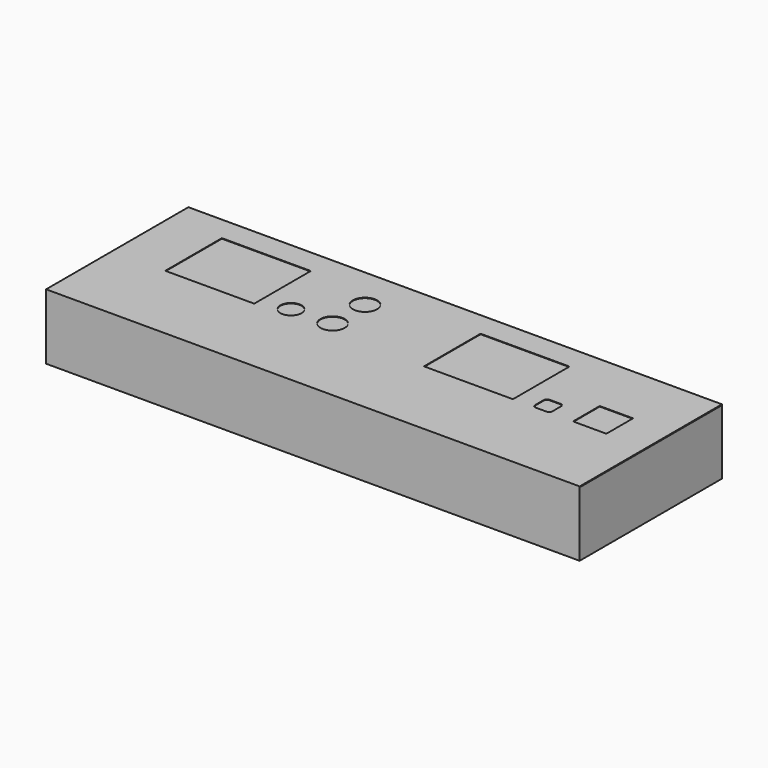
from build123d import *

# Parameters (mm, degrees)
F1_DEPTH = 209.55
F2_W     = 69.85
F2_H     = 55.5625
F2_W_2   = 26.19375
F2_H_2   = 26.19375
F3_DEPTH = 0.4064


# Not quite as in the source:
# - the dataset's text gives a spline's control points without its knots; the knots are read off the source's solid


with BuildPart() as f1:
    # F0 (on Right) → F1 (new body, symmetric)
    with BuildSketch(Plane.YZ):
        Polygon((-139.7, 0), (0, 0), (0, 50.8), (-139.2936, 50.8), (-139.2936, 51.054), (0, 51.054), (0, 51.4604), (-139.7, 51.4604), align=None)
    extrude(amount=F1_DEPTH, both=True)

    # F2 (on face) → F3 (cut, through all)
    with BuildSketch(Plane.XY.offset(51.4604)):
        with Locations((-132.8911783457, -47.0433160888)):
            Rectangle(F2_W, F2_H)
        with Locations((70.3088216543, -47.0433160888)):
            Rectangle(F2_W, F2_H)
        with BuildLine():
            add(Edge.make_bspline(
                [(121.4099132543, -62.0291382888), (120.9689438543, -62.4693964888), (120.7119466543, -63.0892072888), (120.7119466543, -63.7120660888)],
                knots=[1, 1, 1, 1, 2, 2, 2, 2], degree=3))
            Line((120.7119466543, -63.7120660888), (120.7119466543, -72.4433160888))
            add(Edge.make_bspline(
                [(120.7119466543, -72.4433160888), (120.7119466543, -73.0672416888), (120.9689438543, -73.6870016888), (121.4099132543, -74.1272598888)],
                knots=[0, 0, 0, 0, 1, 1, 1, 1], degree=3))
            add(Edge.make_bspline(
                [(121.4099132543, -74.1272598888), (121.8505270543, -74.5682292888), (122.4699822543, -74.8245660888), (123.0931966543, -74.8245660888)],
                knots=[1, 1, 1, 1, 2, 2, 2, 2], degree=3))
            Line((123.0931966543, -74.8245660888), (131.8244466543, -74.8245660888))
            add(Edge.make_bspline(
                [(131.8244466543, -74.8245660888), (132.4483468543, -74.8245660888), (133.0677766543, -74.5682292888), (133.5083904543, -74.1272598888)],
                knots=[0, 0, 0, 0, 1, 1, 1, 1], degree=3))
            add(Edge.make_bspline(
                [(133.5083904543, -74.1272598888), (133.9490042543, -73.6870016888), (134.2056966543, -73.0672416888), (134.2056966543, -72.4433160888)],
                knots=[1, 1, 1, 1, 2, 2, 2, 2], degree=3))
            Line((134.2056966543, -72.4433160888), (134.2056966543, -63.7120660888))
            add(Edge.make_bspline(
                [(134.2056966543, -63.7120660888), (134.2056966543, -63.0892072888), (133.9490042543, -62.4693964888), (133.5083904543, -62.0291382888)],
                knots=[0, 0, 0, 0, 1, 1, 1, 1], degree=3))
            add(Edge.make_bspline(
                [(133.5083904543, -62.0291382888), (133.0677766543, -61.5881688888), (132.4483468543, -61.3308160888), (131.8244466543, -61.3308160888)],
                knots=[1, 1, 1, 1, 2, 2, 2, 2], degree=3))
            Line((131.8244466543, -61.3308160888), (123.0931966543, -61.3308160888))
            add(Edge.make_bspline(
                [(123.0931966543, -61.3308160888), (122.4699822543, -61.3308160888), (121.8505270543, -61.5881688888), (121.4099132543, -62.0291382888)],
                knots=[0, 0, 0, 0, 1, 1, 1, 1], degree=3))
        make_face()
        with Locations((165.5588216543, -61.7276910888)):
            Rectangle(F2_W_2, F2_H_2)
        with BuildLine():
            add(Edge.make_bspline(
                [(-69.8476671457, -60.5980514888), (-71.3907171457, -59.0546712888), (-73.5590643457, -58.1558160888), (-75.7411783457, -58.1558160888)],
                knots=[7, 7, 7, 7, 8, 8, 8, 8], degree=3))
            add(Edge.make_bspline(
                [(-75.7411783457, -58.1558160888), (-77.9229621457, -58.1558160888), (-80.0913093457, -59.0546712888), (-81.6343593457, -60.5980514888)],
                knots=[0, 0, 0, 0, 1, 1, 1, 1], degree=3))
            add(Edge.make_bspline(
                [(-81.6343593457, -60.5980514888), (-83.1771045457, -62.1407712888), (-84.0755533457, -64.3087628888), (-84.0755533457, -66.4901910888), (-84.0755533457, -68.6726606888), (-83.1771045457, -70.8406522888), (-81.6343593457, -72.3840578888)],
                knots=[1, 1, 1, 1, 2, 2, 2, 3, 3, 3, 3], degree=3))
            add(Edge.make_bspline(
                [(-81.6343593457, -72.3840578888), (-80.0913093457, -73.9267776888), (-77.9229621457, -74.8245660888), (-75.7411783457, -74.8245660888), (-73.5590643457, -74.8245660888), (-71.3907171457, -73.9267776888), (-69.8476671457, -72.3840578888)],
                knots=[3, 3, 3, 3, 4, 4, 4, 5, 5, 5, 5], degree=3))
            add(Edge.make_bspline(
                [(-69.8476671457, -72.3840578888), (-68.3049219457, -70.8406522888), (-67.4068033457, -68.6726606888), (-67.4068033457, -66.4901910888), (-67.4068033457, -64.3087628888), (-68.3049219457, -62.1407712888), (-69.8476671457, -60.5980514888)],
                knots=[5, 5, 5, 5, 6, 6, 6, 7, 7, 7, 7], degree=3))
        make_face()
        with BuildLine():
            add(Edge.make_bspline(
                [(-37.2553269457, -58.5644004888), (-39.0188743457, -56.8012086888), (-41.4972793457, -55.7745660888), (-43.9911783457, -55.7745660888)],
                knots=[7, 7, 7, 7, 8, 8, 8, 8], degree=3))
            add(Edge.make_bspline(
                [(-43.9911783457, -55.7745660888), (-46.4843915457, -55.7745660888), (-48.9631521457, -56.8012086888), (-50.7263439457, -58.5644004888)],
                knots=[0, 0, 0, 0, 1, 1, 1, 1], degree=3))
            add(Edge.make_bspline(
                [(-50.7263439457, -58.5644004888), (-52.4895611457, -60.3283034888), (-53.5161783457, -62.8063528888), (-53.5161783457, -65.2995660888), (-53.5161783457, -67.7938206888), (-52.4895611457, -70.2725812888), (-50.7263439457, -72.0350872888)],
                knots=[1, 1, 1, 1, 2, 2, 2, 3, 3, 3, 3], degree=3))
            add(Edge.make_bspline(
                [(-50.7263439457, -72.0350872888), (-48.9631521457, -73.7989648888), (-46.4843915457, -74.8245660888), (-43.9911783457, -74.8245660888), (-41.4972793457, -74.8245660888), (-39.0188743457, -73.7989648888), (-37.2553269457, -72.0350872888)],
                knots=[3, 3, 3, 3, 4, 4, 4, 5, 5, 5, 5], degree=3))
            add(Edge.make_bspline(
                [(-37.2553269457, -72.0350872888), (-35.4921351457, -70.2725812888), (-34.4661783457, -67.7938206888), (-34.4661783457, -65.2995660888), (-34.4661783457, -62.8063528888), (-35.4921351457, -60.3283034888), (-37.2553269457, -58.5644004888)],
                knots=[5, 5, 5, 5, 6, 6, 6, 7, 7, 7, 7], degree=3))
        make_face()
        with BuildLine():
            add(Edge.make_bspline(
                [(-37.2553269457, -26.8144004888), (-39.0188743457, -25.0512086888), (-41.4972793457, -24.0245660888), (-43.9911783457, -24.0245660888)],
                knots=[7, 7, 7, 7, 8, 8, 8, 8], degree=3))
            add(Edge.make_bspline(
                [(-43.9911783457, -24.0245660888), (-46.4843915457, -24.0245660888), (-48.9631521457, -25.0512086888), (-50.7263439457, -26.8144004888)],
                knots=[0, 0, 0, 0, 1, 1, 1, 1], degree=3))
            add(Edge.make_bspline(
                [(-50.7263439457, -26.8144004888), (-52.4895611457, -28.5783034888), (-53.5161783457, -31.0563528888), (-53.5161783457, -33.5495660888), (-53.5161783457, -36.0438206888), (-52.4895611457, -38.5225812888), (-50.7263439457, -40.2850872888)],
                knots=[1, 1, 1, 1, 2, 2, 2, 3, 3, 3, 3], degree=3))
            add(Edge.make_bspline(
                [(-50.7263439457, -40.2850872888), (-48.9631521457, -42.0489648888), (-46.4843915457, -43.0745660888), (-43.9911783457, -43.0745660888), (-41.4972793457, -43.0745660888), (-39.0188743457, -42.0489648888), (-37.2553269457, -40.2850872888)],
                knots=[3, 3, 3, 3, 4, 4, 4, 5, 5, 5, 5], degree=3))
            add(Edge.make_bspline(
                [(-37.2553269457, -40.2850872888), (-35.4921351457, -38.5225812888), (-34.4661783457, -36.0438206888), (-34.4661783457, -33.5495660888), (-34.4661783457, -31.0563528888), (-35.4921351457, -28.5783034888), (-37.2553269457, -26.8144004888)],
                knots=[5, 5, 5, 5, 6, 6, 6, 7, 7, 7, 7], degree=3))
        make_face()
    extrude(amount=-F3_DEPTH, mode=Mode.SUBTRACT)


solid = f1.part
